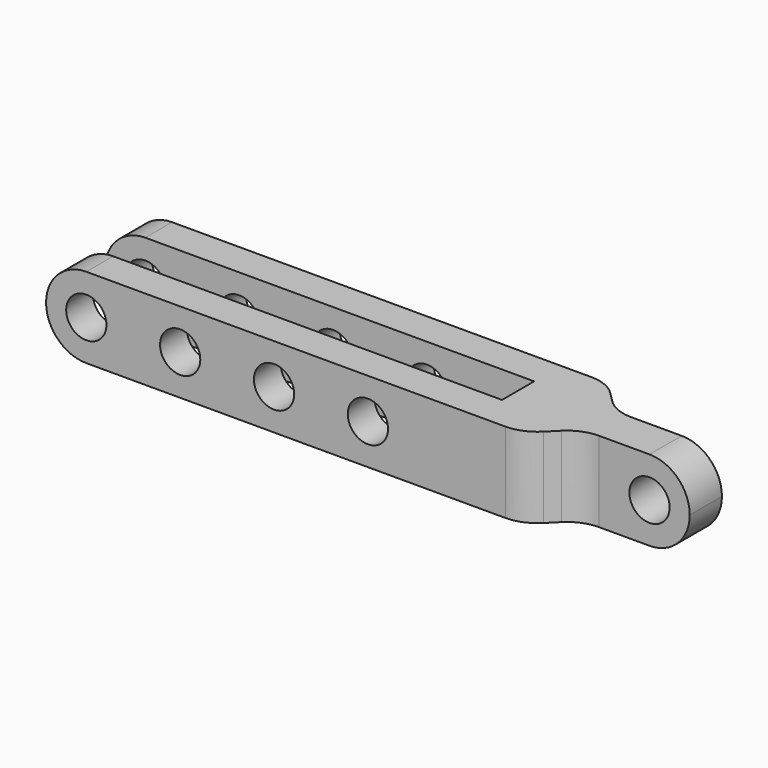
from build123d import *

# Parameters (mm, degrees)
F1_DEPTH = 6
F2_R     = 2.99999
F3_R     = 3
F4_R     = 1.5
F5_R     = 1.5
F6_DEPTH = 25


# Not quite as in the source:
# - a fillet or chamfer is up to 0.001 mm smaller than in the source, because OpenCascade refuses the exact size


with BuildPart() as f1:
    # F0 (on Top) → F1 (new body)
    with BuildSketch(Plane.XY):
        Polygon((15, 1.5), (12.5, 4), (-23, 4), (-23, 1.5), (9, 1.5), (9, -1.5), (-23, -1.5), (-23, -4), (12.5, -4), (15, -1.5), (23, -1.5), (23, 1.5), align=None)
    extrude(amount=F1_DEPTH)

    # F2 (radius 3 in the source; OpenCascade refuses exactly that, so slightly less here)
    f2_edges = [f1.edges().sort_by_distance(p)[0] for p in [
        (-23, -2.75, 6),
        (-23, 2.75, 6),
        (23, 0, 6),
        (23, 0, 0),
        (-23, 2.75, 0),
        (-23, -2.75, 0),
    ]]
    fillet(f2_edges, radius=F2_R)

    # F3
    f3_edges = [f1.edges().sort_by_distance(p)[0] for p in [
        (12.5, 4, 3),
        (15, 1.5, 3),
        (15, -1.5, 3),
        (12.5, -4, 3),
    ]]
    fillet(f3_edges, radius=F3_R)

    # F4 (on face) + F5 (on face) → F6 (cut)
    with BuildSketch(Plane.XZ.offset(4)):
        with Locations((-20, 3)):
            Circle(F4_R)
        with Locations((-13, 3)):
            Circle(F4_R)
        with Locations((-6, 3)):
            Circle(F4_R)
        with Locations((1, 3)):
            Circle(F4_R)
    with BuildSketch(Plane.XZ.offset(1.5)):
        with Locations((20, 3)):
            Circle(F5_R)
    extrude(amount=-F6_DEPTH, mode=Mode.SUBTRACT)


solid = f1.part
